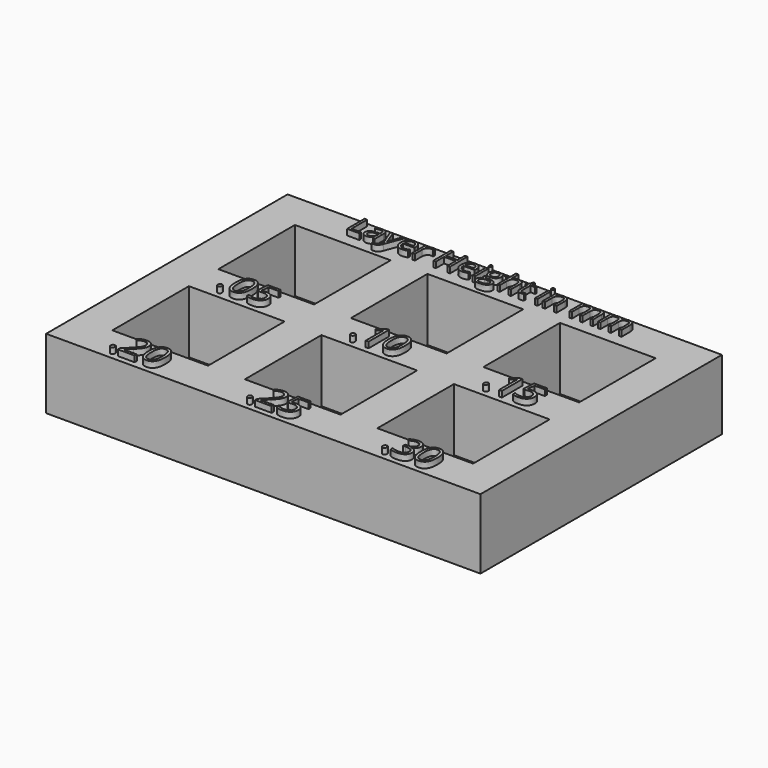
from build123d import *

# Parameters (mm, degrees)
F0_W           = 118
F0_H           = 82
F0_W_2         = 26
F0_H_2         = 26
F1_DEPTH       = 19
F2_DEPTH       = 17
F3_TEXT_SIZE   = 8.3333333333
F3_TEXT_SIZE_2 = 9.7222222222
F4_DEPTH       = 1.6


# Not quite as in the source:
# - a feature names something its author has since deleted; it is built from what else it names
# - Text() gives the source's letters only with a copy of the font that has no kerning and outlines rounded to 1/6400 em; it was checked with that copy


with BuildPart() as f1:
    # F0 (on Top) → F1 (new body)
    with BuildSketch(Plane.XY):
        with Locations((-59, 41)):
            Rectangle(F0_W, F0_H)
        with Locations((-95, 23)):
            Rectangle(F0_W_2, F0_H_2, mode=Mode.SUBTRACT)
        with Locations((-59, 23)):
            Rectangle(F0_W_2, F0_H_2, mode=Mode.SUBTRACT)
        with Locations((-23, 23)):
            Rectangle(F0_W_2, F0_H_2, mode=Mode.SUBTRACT)
        with Locations((-95, 59)):
            Rectangle(F0_W_2, F0_H_2, mode=Mode.SUBTRACT)
        with Locations((-59, 59)):
            Rectangle(F0_W_2, F0_H_2, mode=Mode.SUBTRACT)
        with Locations((-23, 59)):
            Rectangle(F0_W_2, F0_H_2, mode=Mode.SUBTRACT)
        with Locations((-95, 23)):
            Rectangle(F0_W_2, F0_H_2)
        with Locations((-59, 23)):
            Rectangle(F0_W_2, F0_H_2)
        with Locations((-23, 23)):
            Rectangle(F0_W_2, F0_H_2)
        with Locations((-95, 59)):
            Rectangle(F0_W_2, F0_H_2)
        with Locations((-59, 59)):
            Rectangle(F0_W_2, F0_H_2)
        with Locations((-23, 59)):
            Rectangle(F0_W_2, F0_H_2)
    extrude(amount=-F1_DEPTH)

    # F0 (on Top) → F2 (cut)
    with BuildSketch(Plane.XY):
        with Locations((-95, 23)):
            Rectangle(F0_W_2, F0_H_2)
        with Locations((-59, 23)):
            Rectangle(F0_W_2, F0_H_2)
        with Locations((-23, 23)):
            Rectangle(F0_W_2, F0_H_2)
        with Locations((-95, 59)):
            Rectangle(F0_W_2, F0_H_2)
        with Locations((-59, 59)):
            Rectangle(F0_W_2, F0_H_2)
        with Locations((-23, 59)):
            Rectangle(F0_W_2, F0_H_2)
    extrude(amount=-F2_DEPTH, mode=Mode.SUBTRACT)

    # F3 (on face) → F4 (join)
    with BuildSketch(Plane.XY):
        with Locations((-97.1377938986, 75.131208688)):
            Text('Layer Height in mm', F3_TEXT_SIZE, font='Open Sans', text_align=(TextAlign.LEFT, TextAlign.BOTTOM))
        with Locations((-102.4734005332, 37.5)):
            Text('.05', F3_TEXT_SIZE_2, font='Open Sans', text_align=(TextAlign.LEFT, TextAlign.BOTTOM))
        with Locations((-66.3718208671, 37.5)):
            Text('.10', F3_TEXT_SIZE_2, font='Open Sans', text_align=(TextAlign.LEFT, TextAlign.BOTTOM))
        with Locations((-30.1507469267, 37.5)):
            Text('.15', F3_TEXT_SIZE_2, font='Open Sans', text_align=(TextAlign.LEFT, TextAlign.BOTTOM))
        with Locations((-102.7613654733, 1.5)):
            Text('.20', F3_TEXT_SIZE_2, font='Open Sans', text_align=(TextAlign.LEFT, TextAlign.BOTTOM))
        with Locations((-65.526846313, 1.5)):
            Text('.25', F3_TEXT_SIZE_2, font='Open Sans', text_align=(TextAlign.LEFT, TextAlign.BOTTOM))
        with Locations((-28.8658291101, 1.5)):
            Text('.30', F3_TEXT_SIZE_2, font='Open Sans', text_align=(TextAlign.LEFT, TextAlign.BOTTOM))
    extrude(amount=F4_DEPTH)


solid = f1.part
